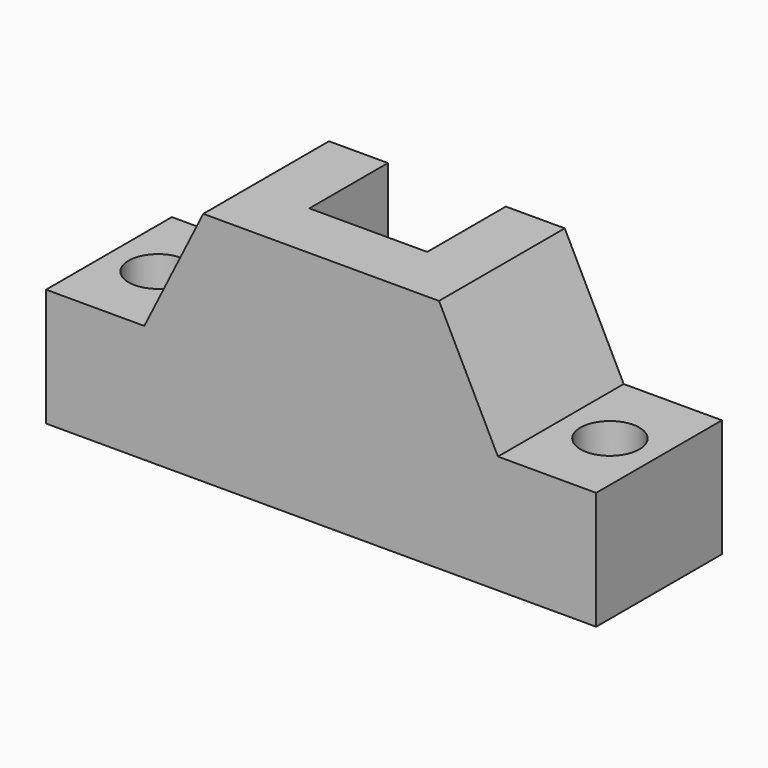
from build123d import *

# Parameters (mm, degrees)
F1_DEPTH    = 40
F2_W        = 30
F2_H        = 45
F3_DEPTH    = 25
F4_T4_DEPTH = 30
F5_R        = 7.5
F6_DEPTH    = 30


# Not quite as in the source:
# - a fillet or chamfer that OpenCascade refuses, or shapes differently, is made with other operations: its cross-section is extruded or revolved along the edge and cut away or added


with BuildPart() as f1:
    # F0 (on Front) → F1 (new body)
    with BuildSketch(Plane.XZ):
        Polygon((0, 30), (0, 0), (140, 0), (140, 30), (115, 30), (100, 60), (85, 60), (55, 60), (40, 60), (25, 30), align=None)
    extrude(amount=F1_DEPTH)

    # F2 (on Front) → F3 (cut)
    with BuildSketch(Plane.XZ):
        with Locations((70, 37.5)):
            Rectangle(F2_W, F2_H)
    extrude(amount=F3_DEPTH, mode=Mode.SUBTRACT)

    # F4: chamfer of 45 x 25.9807621135 on 1 edges, made by hand


with BuildPart() as f4_tool2:
    # F4_s3 → F4_t4 (new body)
    with BuildSketch(Plane.YZ.offset(55)):
        Polygon((0.9807621135, 15), (-25, 60), (-25, 15), align=None)
    extrude(amount=F4_T4_DEPTH)

    split(bisect_by=Plane.XZ, keep=Keep.TOP)

    split(bisect_by=Plane.XY.offset(60), keep=Keep.BOTTOM)


with BuildPart() as f1_1:
    add(f1.part)

    # F4_t1: union F4_tool2
    add(f4_tool2.part)

    # F5 (on Top) → F6 (cut)
    with BuildSketch(Plane.XY):
        with Locations((127.5, -20)):
            Circle(F5_R)
        with BuildLine():
            ThreePointArc((12.5, -12.5), (7.1966991411, -25.3033008589), (20, -20))
            ThreePointArc((20, -20), (17.8033008589, -14.6966991411), (12.5, -12.5))
        make_face()
    extrude(amount=F6_DEPTH, mode=Mode.SUBTRACT)


solid = f1_1.part
